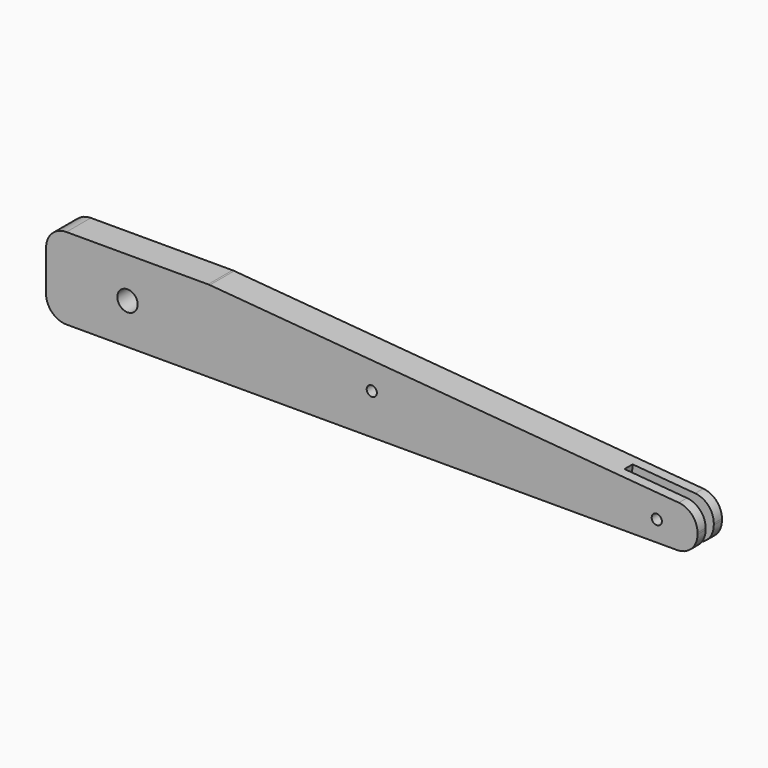
from build123d import *

# Parameters (mm, degrees)
F0_W          = 406.4
F0_H          = 50.8
F0_R          = 3.175
F1_DEPTH      = 19.05
F2_SIZE2      = 25.4
F2_SIZE       = 304.8
F3_R          = 6.35
F4_DEPTH      = 19.051
F5_R          = 3.175
F6_DEPTH      = 19.051
F7_W          = 50.8
F7_H          = 6.35
F8_DEPTH      = 59.062945272
F9_W          = 6.35
F9_H          = 25.4
F10_DEPTH     = 2.54
F11_T1_DEPTH  = 82.55
F11_T3_DEPTH  = 69.85
F11_T5_DEPTH  = 69.85
F11_T7_DEPTH  = 64.7784379794
F11_T9_DEPTH  = 64.7784379794
F11_T11_DEPTH = 21.6912557533


# Not quite as in the source:
# - a fillet or chamfer that OpenCascade refuses, or shapes differently, is made with other operations: its cross-section is extruded or revolved along the edge and cut away or added


with BuildPart() as f1:
    # F0 (on Front) → F1 (new body)
    with BuildSketch(Plane.XZ):
        Rectangle(F0_W, F0_H)
        Circle(F0_R, mode=Mode.SUBTRACT)
    extrude(amount=F1_DEPTH)

    # F2
    f2_edges = [f1.edges().sort_by_distance(p)[0] for p in [
        (203.2, -9.525, 25.4),
    ]]
    f2_side = f1.faces().sort_by_distance((0, -9.525, 25.4))[0]
    chamfer(f2_edges, length=F2_SIZE, length2=F2_SIZE2, reference=f2_side)

    # F3 (on face) → F4 (cut, through all)
    with BuildSketch(Plane.XZ.offset(19.05)):
        with Locations((-152.4, 0)):
            Circle(F3_R)
    extrude(amount=-F4_DEPTH, mode=Mode.SUBTRACT)

    # F5 (on face) → F6 (cut, through all)
    with BuildSketch(Plane.XZ.offset(19.05)):
        with Locations((177.8, -12.7)):
            Circle(F5_R)
    extrude(amount=-F6_DEPTH, mode=Mode.SUBTRACT)

    # F7 (on face) → F8 (cut, through all)
    with BuildSketch(Plane(origin=(1.4013793103, 0, 16.8165517241), x_dir=(0.9965457582, 0, -0.0830454799), z_dir=(0.0830454799, 0, 0.9965457582))):
        with Locations((177.0980980754, -9.525)):
            Rectangle(F7_W, F7_H)
    extrude(amount=-F8_DEPTH, mode=Mode.SUBTRACT)

    # F9 (on face) → F10 (cut)
    with BuildSketch(Plane.YZ.offset(203.2)):
        with Locations((-9.525, -12.7)):
            Rectangle(F9_W, F9_H)
    extrude(amount=-F10_DEPTH, mode=Mode.SUBTRACT)

    # F11: fillet of radius 12.7 on 7 edges, made by hand

    # F11_s2 → F11_t1 (cut)
    with BuildSketch(Plane.XZ.offset(-31.75)):
        with BuildLine():
            ThreePointArc((-190.5, 25.4), (-199.4802561211, 21.6802561211), (-203.2, 12.7))
            Line((-203.2, 12.7), (-203.2, 25.4))
            Line((-203.2, 25.4), (-190.5, 25.4))
        make_face()
        with BuildLine():
            ThreePointArc((-190.5, -25.4), (-199.4802561211, -21.6802561211), (-203.2, -12.7))
            Line((-203.2, -12.7), (-203.2, -25.4))
            Line((-203.2, -25.4), (-190.5, -25.4))
        make_face()
    extrude(amount=F11_T1_DEPTH, mode=Mode.SUBTRACT)

    # F11_s4 → F11_t3 (cut)
    with BuildSketch(Plane.XZ.offset(-19.05)):
        with BuildLine():
            ThreePointArc((190.5, -25.4), (199.4802561211, -21.6802561211), (203.2, -12.7))
            Line((203.2, -12.7), (203.2, -25.4))
            Line((203.2, -25.4), (190.5, -25.4))
        make_face()
    extrude(amount=F11_T3_DEPTH, mode=Mode.SUBTRACT)

    # F11_s6 → F11_t5 (cut)
    with BuildSketch(Plane.XZ.offset(-31.75)):
        with BuildLine():
            ThreePointArc((203.2, -12.7), (199.4802561211, -21.6802561211), (190.5, -25.4))
            Line((190.5, -25.4), (203.2, -25.4))
            Line((203.2, -25.4), (203.2, -12.7))
        make_face()
    extrude(amount=F11_T5_DEPTH, mode=Mode.SUBTRACT)

    # F11_s8 → F11_t7 (cut)
    with BuildSketch(Plane.XZ.offset(-29.2142189897)):
        with BuildLine():
            ThreePointArc((203.2, -11.6856875959), (199.8457050415, -3.0863970858), (191.5546775941, 0.9704435338))
            Line((191.5546775941, 0.9704435338), (203.2, 0))
            Line((203.2, 0), (203.2, -11.6856875959))
        make_face()
    extrude(amount=F11_T7_DEPTH, mode=Mode.SUBTRACT)

    # F11_s10 → F11_t9 (cut)
    with BuildSketch(Plane.XZ.offset(-16.5142189897)):
        with BuildLine():
            ThreePointArc((203.2, -11.6856875959), (199.8457050415, -3.0863970858), (191.5546775941, 0.9704435338))
            Line((191.5546775941, 0.9704435338), (203.2, 0))
            Line((203.2, 0), (203.2, -11.6856875959))
        make_face()
    extrude(amount=F11_T9_DEPTH, mode=Mode.SUBTRACT)

    # F11_s12 → F11_t11 (cut)
    with BuildSketch(Plane.XZ.offset(-1.3206278767)):
        with BuildLine():
            ThreePointArc((-102.1282511507, 25.4), (-101.6004563739, 25.3890280429), (-101.0735735565, 25.3561311297))
            Line((-101.0735735565, 25.3561311297), (-101.6, 25.4))
            Line((-101.6, 25.4), (-102.1282511507, 25.4))
        make_face()
    extrude(amount=F11_T11_DEPTH, mode=Mode.SUBTRACT)


solid = f1.part
